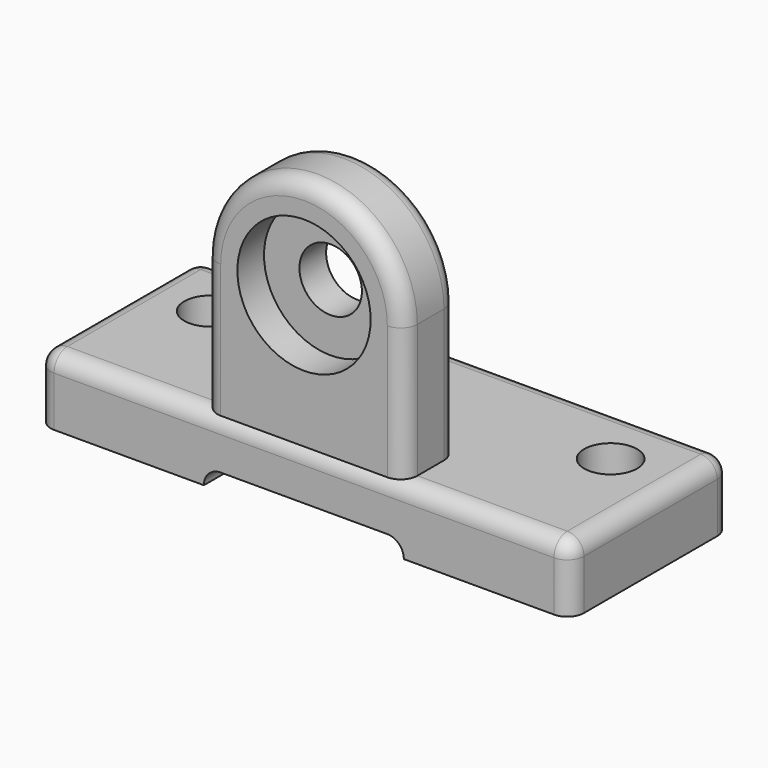
from build123d import *

# Parameters (mm, degrees)
F0_W           = 101.6
F0_H           = 38.1
F1_DEPTH       = 12.7
F3_DEPTH       = 12.7
F5_D           = 11.90625
F5_CBORE_D     = 25.4
F5_CBORE_DEPTH = 6.35
F6_W           = 38.1
F6_H           = 3.175
F7_DEPTH       = 38.101
F9_D           = 10.0838
F10_D          = 10.0838
F11_R          = 3.175
F12_R          = 3.17499
F12_2_R        = 3.17499


# Not quite as in the source:
# - a fillet or chamfer is up to 0.001 mm smaller than in the source, because OpenCascade refuses the exact size
# - a length typed as a fraction of an inch, garbled in the dataset ("3 / 203.2 mm" for 3/8 in), is restored


with BuildPart() as f1:
    # F0 (on Top) → F1 (new body)
    with BuildSketch(Plane.XY):
        Rectangle(F0_W, F0_H)
    extrude(amount=F1_DEPTH)

    # F6 (on face) → F7 (cut, through all)
    with BuildSketch(Plane(origin=(0, 19.05, 0), x_dir=(-1, 0, 0), z_dir=(0, 1, 0))):
        with Locations((0.028450042, 1.5875)):
            Rectangle(F6_W, F6_H)
    extrude(amount=-F7_DEPTH, mode=Mode.SUBTRACT)

    # F9 (through all)
    with Locations(Plane.XY.offset(12.7)):
        with Locations((-38.1, 6.35)):
            Hole(F9_D / 2)

    # F10 (through all)
    with Locations(Plane.XY.offset(12.7)):
        with Locations((38.1, 6.35)):
            Hole(F10_D / 2)

    # F11
    f11_edges = [f1.edges().sort_by_distance(p)[0] for p in [
        (50.8, -19.05, 6.35),
        (50.8, 19.05, 6.35),
        (-50.8, -19.05, 6.35),
        (-50.8, 19.05, 6.35),
    ]]
    fillet(f11_edges, radius=F11_R)

    # F12 (radius 3.175 in the source; OpenCascade refuses exactly that, so slightly less here)
    f12_edges = [f1.edges().sort_by_distance(p)[0] for p in [
        (19.02155, 0, 3.175),
        (-19.07845, 0, 3.175),
        (0, 19.05, 12.7),
    ]]
    fillet(f12_edges, radius=F12_R)


with BuildPart() as f3:
    # F2 (on face) → F3 (new body)
    with BuildSketch(Plane.XZ.offset(19.05)):
        with BuildLine():
            Line((-19.05, 38.1), (-19.05, 12.7))
            Line((-19.05, 12.7), (19.05, 12.7))
            Line((19.05, 12.7), (19.05, 38.1))
            ThreePointArc((19.05, 38.1), (0, 57.15), (-19.05, 38.1))
        make_face()
    extrude(amount=-F3_DEPTH)

    # F5 (through all)
    with Locations(Plane.XZ.offset(19.05)):
        with Locations((0, 38.1)):
            CounterBoreHole(F5_D / 2, F5_CBORE_D / 2, F5_CBORE_DEPTH)

    # F12#2 (radius 3.175 in the source; OpenCascade refuses exactly that, so slightly less here)
    f12_2_edges = [f3.edges().sort_by_distance(p)[0] for p in [
        (0, -19.05, 57.15),
        (0, -6.35, 57.15),
        (19.05, -19.05, 25.4),
        (19.05, -6.35, 25.4),
        (-19.05, -19.05, 25.4),
        (-19.05, -6.35, 25.4),
    ]]
    fillet(f12_2_edges, radius=F12_2_R)


solid = Compound([f1.part, f3.part])
